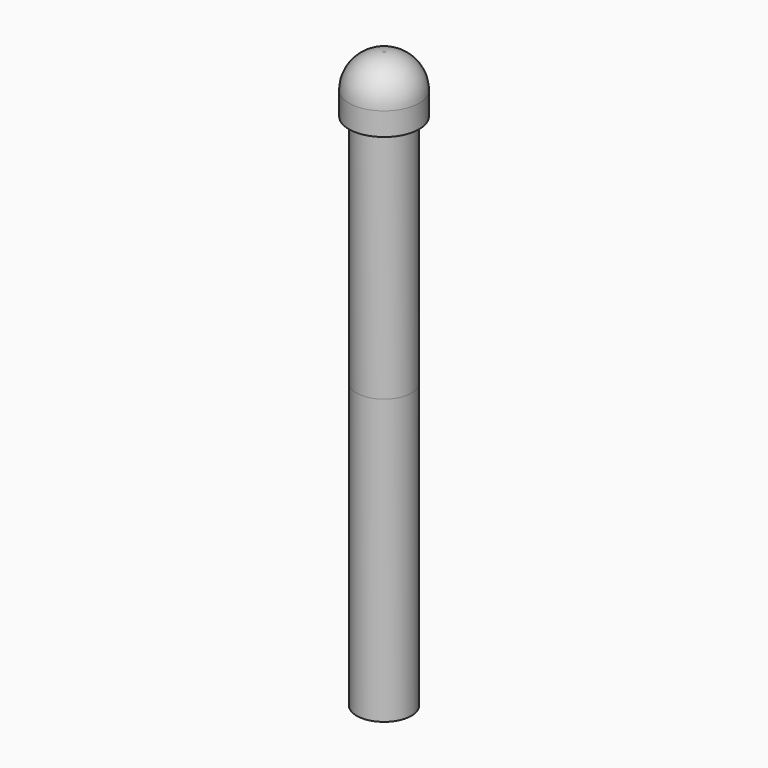
from build123d import *

# Parameters (mm, degrees)
F0_R     = 1.8364004546
F1_DEPTH = 15.748
F2_R     = 2.355472205
F2_R_2   = 1.8364004546
F3_DEPTH = 3.81
F4_R     = 2.2688779059
F5_R     = 1.8364004546
F6_DEPTH = 19.05


with BuildPart() as f1:
    # F0 (on Top) → F1 (new body)
    with BuildSketch(Plane.XY):
        Circle(F0_R)
    extrude(amount=F1_DEPTH)


with BuildPart() as f3:
    # F2 (on face) → F3 (new body)
    with BuildSketch(Plane.XY.offset(15.748)):
        Circle(F2_R)
        Circle(F2_R_2, mode=Mode.SUBTRACT)
        Circle(F2_R_2)
    extrude(amount=F3_DEPTH)

    # F4
    f4_edges = [f3.edges().sort_by_distance(p)[0] for p in [
        (-2.355472, 0, 19.558),
    ]]
    fillet(f4_edges, radius=F4_R)


with BuildPart() as f6:
    # F5 (on face) → F6 (new body)
    with BuildSketch(Plane(origin=(0, 0, 0), x_dir=(1, 0, 0), z_dir=(0, 0, -1))):
        Circle(F5_R)
    extrude(amount=F6_DEPTH)


solid = Compound([f1.part, f3.part, f6.part])
